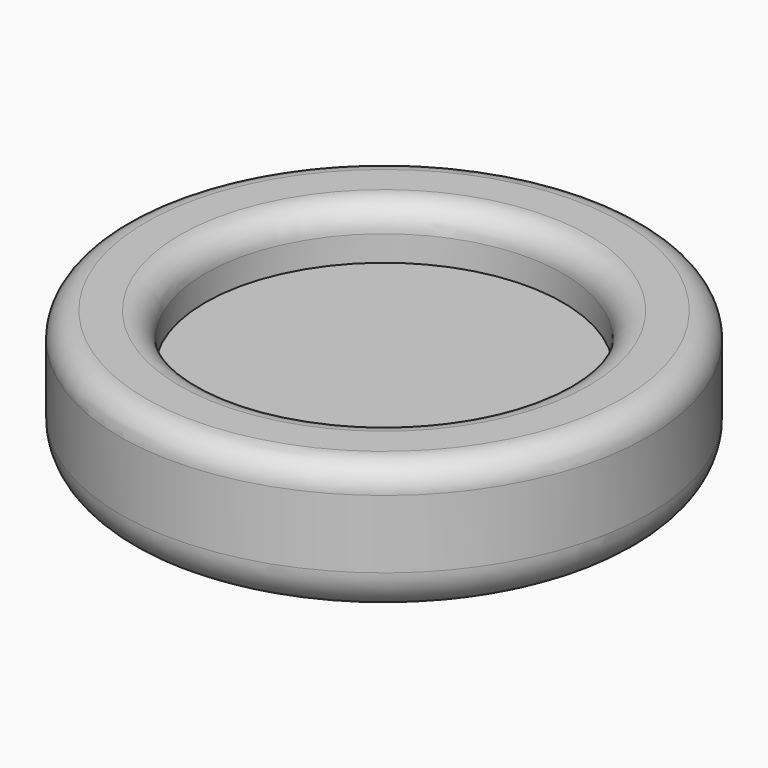
from build123d import *

# Parameters (mm, degrees)
F0_R     = 15.5
F1_DEPTH = 8
F2_T     = -5
F3_R     = 1.5
F4_R     = 2.5


with BuildPart() as f1:
    # F0 (on Top) → F1 (new body)
    with BuildSketch(Plane.XY):
        with Locations((-13.3484182879, 0)):
            Circle(F0_R)
    extrude(amount=F1_DEPTH)

    # F2
    f2_openings = [f1.faces().sort_by_distance(p)[0] for p in [
        (-13.348418, 0, 8),
    ]]
    offset(amount=F2_T, openings=f2_openings)

    # F3
    f3_edges = [f1.edges().sort_by_distance(p)[0] for p in [
        (-28.848418, 0, 8),
        (-23.848418, 0, 8),
    ]]
    fillet(f3_edges, radius=F3_R)

    # F4
    f4_edges = [f1.edges().sort_by_distance(p)[0] for p in [
        (-28.848418, 0, 0),
    ]]
    fillet(f4_edges, radius=F4_R)


solid = f1.part
